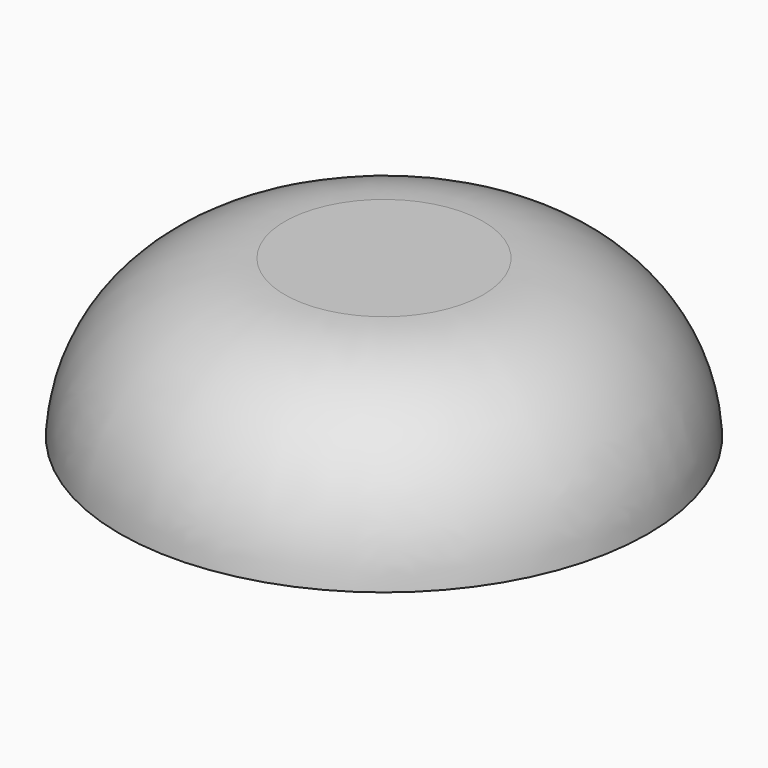
from build123d import *

# Parameters (mm, degrees)
F0_R     = 3.2
F1_DEPTH = 1.9


# Not quite as in the source:
# - a fillet or chamfer that OpenCascade refuses, or shapes differently, is made with other operations: its cross-section is extruded or revolved along the edge and cut away or added


with BuildPart() as f1:
    # F0 (on Top) → F1 (new body)
    with BuildSketch(Plane.XY):
        Circle(F0_R)
    extrude(amount=F1_DEPTH)

    # F2: fillet of radius 2 on 1 edges, made by hand

    # F2_s1 → F2_t2 (revolve, cut)
    with BuildSketch(Plane.XZ):
        with BuildLine():
            ThreePointArc((3.2, 0), (2.5809064397, 1.3491376746), (1.2025015645, 1.9))
            Line((1.2025015645, 1.9), (3.2, 1.9))
            Line((3.2, 1.9), (3.2, 0))
        make_face()
    revolve(axis=Axis((0, 0, 1.9), (0, 0, 1)), mode=Mode.SUBTRACT)


solid = f1.part
